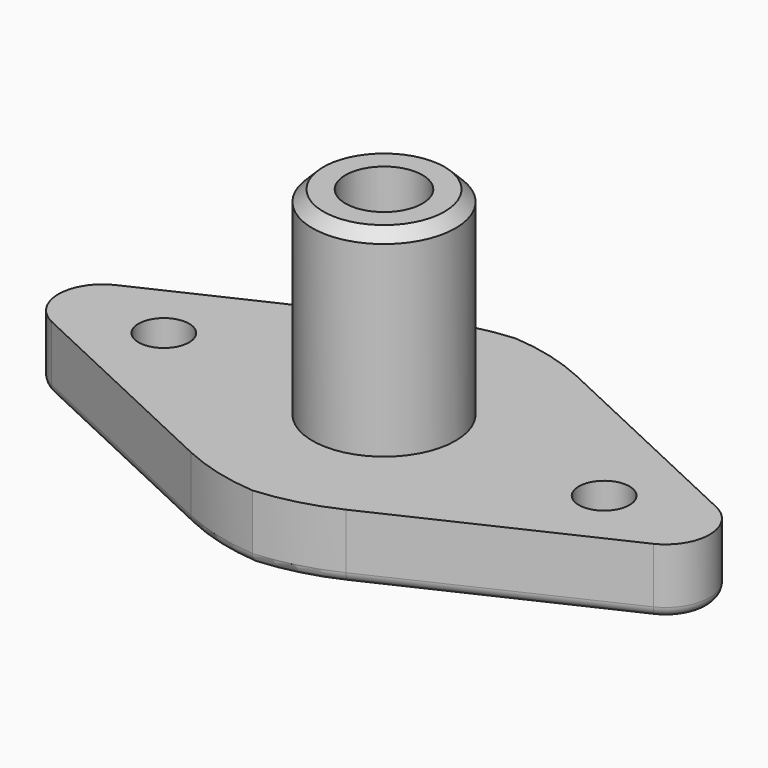
from build123d import *

# Parameters (mm, degrees)
F1_DEPTH      = 3
F2_T1_DEPTH   = 24.3364797517
F3_T1_DEPTH   = 14.1373136471
F4_R          = 3.25
F5_DEPTH      = 9
F6_R          = 1.75
F7_DEPTH      = 12.001
F8_SIZE       = 0.5
F4_R_2        = 1.15
F9_DEPTH      = 3.001
F10_SIZE      = 1
F11_T1_DEPTH  = 11.2158433332
F11_T3_DEPTH  = 11.2158433332
F11_T5_DEPTH  = 11.2158433332
F11_T7_DEPTH  = 11.2158433332
F11_T10_ANGLE = 127.4788590763
F11_T12_ANGLE = 42.4709850422
F11_T14_ANGLE = 42.4709850422
F11_T16_ANGLE = 42.4709850422
F11_T18_ANGLE = 42.4709850422
F11_T20_ANGLE = 127.4788590763


# Not quite as in the source:
# - a fillet or chamfer that OpenCascade refuses, or shapes differently, is made with other operations: its cross-section is extruded or revolved along the edge and cut away or added


with BuildPart() as f1:
    # F0 (on Top) → F1 (new body)
    with BuildSketch(Plane.XY):
        Polygon((-1.5, 7.5), (-17.5, 0), (-1.5, -7.5), (1.5, -7.5), (17.5, 0), (1.5, 7.5), align=None)
    extrude(amount=F1_DEPTH)

    # F2: fillet of radius 2 on 2 edges, made by hand

    # F2_s2 → F2_t1 (cut)
    with BuildSketch(Plane.XY.offset(-10.6682398759)):
        with BuildLine():
            ThreePointArc((-13.6363085399, 1.8115471368), (-14.7878407874, 0), (-13.6363085399, -1.8115471368))
            Line((-13.6363085399, -1.8115471368), (-13.7212248119, -1.9927018505))
            ThreePointArc((-13.7212248119, -1.9927018505), (-15.6529856552, -1.0867471903), (-17.584916272, -0.1811547137))
            Line((-17.584916272, -0.1811547137), (-17.584916272, 0.1811547137))
            ThreePointArc((-17.584916272, 0.1811547137), (-15.6529856552, 1.0867471903), (-13.7212248119, 1.9927018505))
            Line((-13.7212248119, 1.9927018505), (-13.6363085399, 1.8115471368))
        make_face()
        with BuildLine():
            ThreePointArc((13.6363085399, -1.8115471368), (14.7878407874, 0), (13.6363085399, 1.8115471368))
            Line((13.6363085399, 1.8115471368), (13.7212248119, 1.9927018505))
            ThreePointArc((13.7212248119, 1.9927018505), (15.6529856552, 1.0867471903), (17.584916272, 0.1811547137))
            Line((17.584916272, 0.1811547137), (17.584916272, -0.1811547137))
            ThreePointArc((17.584916272, -0.1811547137), (15.6529856552, -1.0867471903), (13.7212248119, -1.9927018505))
            Line((13.7212248119, -1.9927018505), (13.6363085399, -1.8115471368))
        make_face()
    extrude(amount=F2_T1_DEPTH, mode=Mode.SUBTRACT)

    # F3: fillet of radius 10 on 4 edges, made by hand

    # F3_s2 → F3_t1 (cut)
    with BuildSketch(Plane.XY.offset(-5.5686568236)):
        with BuildLine():
            ThreePointArc((-3.5168760329, 6.5545893596), (-1.4467160125, 7.2607861772), (0.7274627294, 7.5))
            Line((0.7274627294, 7.5), (-1.5, 7.5))
            Line((-1.5, 7.5), (-3.5168760329, 6.5545893596))
        make_face()
        with BuildLine():
            ThreePointArc((-0.7274627294, 7.5), (1.4467160125, 7.2607861772), (3.5168760329, 6.5545893596))
            Line((3.5168760329, 6.5545893596), (1.5, 7.5))
            Line((1.5, 7.5), (-0.7274627294, 7.5))
        make_face()
        with BuildLine():
            ThreePointArc((3.5168760329, -6.5545893596), (1.4467160125, -7.2607861772), (-0.7274627294, -7.5))
            Line((-0.7274627294, -7.5), (1.5, -7.5))
            Line((1.5, -7.5), (3.5168760329, -6.5545893596))
        make_face()
        with BuildLine():
            ThreePointArc((0.7274627294, -7.5), (-1.4467160125, -7.2607861772), (-3.5168760329, -6.5545893596))
            Line((-3.5168760329, -6.5545893596), (-1.5, -7.5))
            Line((-1.5, -7.5), (0.7274627294, -7.5))
        make_face()
    extrude(amount=F3_T1_DEPTH, mode=Mode.SUBTRACT)

    # F4 (on face) → F5 (join)
    with BuildSketch(Plane.XY.offset(3)):
        Circle(F4_R)
    extrude(amount=F5_DEPTH)

    # F6 (on face) → F7 (cut, through all)
    with BuildSketch(Plane.XY.offset(12)):
        Circle(F6_R)
    extrude(amount=-F7_DEPTH, mode=Mode.SUBTRACT)

    # F8
    f8_edges = [f1.edges().sort_by_distance(p)[0] for p in [
        (-3.25, 0, 12),
    ]]
    chamfer(f8_edges, length=F8_SIZE)

    # F4 (on face) → F9 (cut, through all)
    with BuildSketch(Plane.XY.offset(3)):
        with Locations((-10, 0)):
            Circle(F4_R_2)
        with Locations((10, 0)):
            Circle(F4_R_2)
    extrude(amount=-F9_DEPTH, mode=Mode.SUBTRACT)

    # F10
    f10_edges = [f1.edges().sort_by_distance(p)[0] for p in [
        (-11.15, 0, 0),
        (8.85, 0, 0),
    ]]
    chamfer(f10_edges, length=F10_SIZE)

    # F11: fillet of radius 0.5 on 10 edges, made by hand

    # F11_s2 → F11_t1 (cut)
    with BuildSketch(Plane(origin=(-10.5198395857, 4.9311748058, 0), x_dir=(0, 0, 1), z_dir=(0.905458936, -0.4244338762, 0))):
        with BuildLine():
            ThreePointArc((-0.0004, 6.9266271486), (0.1464466094, 7.2811462246), (0.5009656854, 7.427992834))
            Line((0.5009656854, 7.427992834), (0.5009656854, 7.4781294026))
            ThreePointArc((0.5009656854, 7.4781294026), (0.2504828427, 7.4777294026), (0, 7.4777294026))
            Line((0, 7.4777294026), (-0.0501365685, 7.427592834))
            ThreePointArc((-0.0501365685, 7.427592834), (-0.0501365685, 7.1771099913), (-0.0505365685, 6.9266271486))
            Line((-0.0505365685, 6.9266271486), (-0.0004, 6.9266271486))
        make_face()
    extrude(amount=F11_T1_DEPTH, mode=Mode.SUBTRACT)

    # F11_s4 → F11_t3 (cut)
    with BuildSketch(Plane(origin=(0.3643540153, 0.1707909447, 0), x_dir=(0, 0, 1), z_dir=(0.905458936, 0.4244338762, 0))):
        with BuildLine():
            ThreePointArc((-0.0004, 6.9266271486), (0.1464466094, 7.2811462246), (0.5009656854, 7.427992834))
            Line((0.5009656854, 7.427992834), (0.5009656854, 7.4781294026))
            ThreePointArc((0.5009656854, 7.4781294026), (0.2504828427, 7.4777294026), (0, 7.4777294026))
            Line((0, 7.4777294026), (-0.0501365685, 7.427592834))
            ThreePointArc((-0.0501365685, 7.427592834), (-0.0501365685, 7.1771099913), (-0.0505365685, 6.9266271486))
            Line((-0.0505365685, 6.9266271486), (-0.0004, 6.9266271486))
        make_face()
    extrude(amount=F11_T3_DEPTH, mode=Mode.SUBTRACT)

    # F11_s6 → F11_t5 (cut)
    with BuildSketch(Plane(origin=(10.5198395857, -4.9311748058, 0), x_dir=(0, 0, 1), z_dir=(-0.905458936, 0.4244338762, 0))):
        with BuildLine():
            ThreePointArc((-0.0004, 6.9266271486), (0.1464466094, 7.2811462246), (0.5009656854, 7.427992834))
            Line((0.5009656854, 7.427992834), (0.5009656854, 7.4781294026))
            ThreePointArc((0.5009656854, 7.4781294026), (0.2504828427, 7.4777294026), (0, 7.4777294026))
            Line((0, 7.4777294026), (-0.0501365685, 7.427592834))
            ThreePointArc((-0.0501365685, 7.427592834), (-0.0501365685, 7.1771099913), (-0.0505365685, 6.9266271486))
            Line((-0.0505365685, 6.9266271486), (-0.0004, 6.9266271486))
        make_face()
    extrude(amount=F11_T5_DEPTH, mode=Mode.SUBTRACT)

    # F11_s8 → F11_t7 (cut)
    with BuildSketch(Plane(origin=(-0.3643540153, -0.1707909447, 0), x_dir=(0, 0, 1), z_dir=(-0.905458936, -0.4244338762, 0))):
        with BuildLine():
            ThreePointArc((-0.0004, 6.9266271486), (0.1464466094, 7.2811462246), (0.5009656854, 7.427992834))
            Line((0.5009656854, 7.427992834), (0.5009656854, 7.4781294026))
            ThreePointArc((0.5009656854, 7.4781294026), (0.2504828427, 7.4777294026), (0, 7.4777294026))
            Line((0, 7.4777294026), (-0.0501365685, 7.427592834))
            ThreePointArc((-0.0501365685, 7.427592834), (-0.0501365685, 7.1771099913), (-0.0505365685, 6.9266271486))
            Line((-0.0505365685, 6.9266271486), (-0.0004, 6.9266271486))
        make_face()
    extrude(amount=F11_T7_DEPTH, mode=Mode.SUBTRACT)

    # F11_s9 → F11_t10 (revolve, cut)
    with BuildSketch(Plane(origin=(10.283861632, -5.0737982035, 0), x_dir=(0, 0, 1), z_dir=(-0.8967911287, 0.4424541462, 0))):
        with BuildLine():
            ThreePointArc((-0.0004, 7.157454968), (0.1464466094, 7.511974044), (0.5009656854, 7.6588206534))
            Line((0.5009656854, 7.6588206534), (0.5009656854, 7.708957222))
            ThreePointArc((0.5009656854, 7.708957222), (0.2504828427, 7.708557222), (0, 7.708557222))
            Line((0, 7.708557222), (-0.0501365685, 7.6584206534))
            ThreePointArc((-0.0501365685, 7.6584206534), (-0.0501365685, 7.4079378107), (-0.0505365685, 7.157454968))
            Line((-0.0505365685, 7.157454968), (-0.0004, 7.157454968))
        make_face()
    revolve(axis=Axis((12.7871458195, 0, 0), (0, 0, -1)), revolution_arc=F11_T10_ANGLE, mode=Mode.SUBTRACT)

    # F11_s11 → F11_t12 (revolve, cut)
    with BuildSketch(Plane(origin=(-1.3745464916, -0.429601751, 0), x_dir=(0, 0, 1), z_dir=(-0.9544689122, -0.2983104016, 0))):
        with BuildLine():
            ThreePointArc((-0.0004, 7.3298717335), (0.1464466094, 7.6843908095), (0.5009656854, 7.8312374189))
            Line((0.5009656854, 7.8312374189), (0.5009656854, 7.8813739874))
            ThreePointArc((0.5009656854, 7.8813739874), (0.2504828427, 7.8809739874), (0, 7.8809739874))
            Line((0, 7.8809739874), (-0.0501365685, 7.8308374189))
            ThreePointArc((-0.0501365685, 7.8308374189), (-0.0501365685, 7.5803545762), (-0.0505365685, 7.3298717335))
            Line((-0.0505365685, 7.3298717335), (-0.0004, 7.3298717335))
        make_face()
    revolve(axis=Axis((-0.72746273, -2.5000000027, 0), (0, 0, -1)), revolution_arc=F11_T12_ANGLE, mode=Mode.SUBTRACT)

    # F11_s13 → F11_t14 (revolve, cut)
    with BuildSketch(Plane(origin=(-0.3643540157, -0.1707909448, 0), x_dir=(0, 0, 1), z_dir=(-0.905458936, -0.4244338762, 0))):
        with BuildLine():
            ThreePointArc((-0.0004, 6.9266271486), (0.1464466094, 7.2811462246), (0.5009656854, 7.427992834))
            Line((0.5009656854, 7.427992834), (0.5009656854, 7.4781294026))
            ThreePointArc((0.5009656854, 7.4781294026), (0.2504828427, 7.4777294026), (0, 7.4777294026))
            Line((0, 7.4777294026), (-0.0501365685, 7.427592834))
            ThreePointArc((-0.0501365685, 7.427592834), (-0.0501365685, 7.1771099913), (-0.0505365685, 6.9266271486))
            Line((-0.0505365685, 6.9266271486), (-0.0004, 6.9266271486))
        make_face()
    revolve(axis=Axis((0.72746273, -2.5000000027, 0), (0, 0, -1)), revolution_arc=F11_T14_ANGLE, mode=Mode.SUBTRACT)

    # F11_s15 → F11_t16 (revolve, cut)
    with BuildSketch(Plane(origin=(0.3643540157, 0.1707909448, 0), x_dir=(0, 0, 1), z_dir=(0.905458936, 0.4244338762, 0))):
        with BuildLine():
            ThreePointArc((-0.0004, 6.9266271486), (0.1464466094, 7.2811462246), (0.5009656854, 7.427992834))
            Line((0.5009656854, 7.427992834), (0.5009656854, 7.4781294026))
            ThreePointArc((0.5009656854, 7.4781294026), (0.2504828427, 7.4777294026), (0, 7.4777294026))
            Line((0, 7.4777294026), (-0.0501365685, 7.427592834))
            ThreePointArc((-0.0501365685, 7.427592834), (-0.0501365685, 7.1771099913), (-0.0505365685, 6.9266271486))
            Line((-0.0505365685, 6.9266271486), (-0.0004, 6.9266271486))
        make_face()
    revolve(axis=Axis((-0.72746273, 2.5000000027, 0), (0, 0, -1)), revolution_arc=F11_T16_ANGLE, mode=Mode.SUBTRACT)

    # F11_s17 → F11_t18 (revolve, cut)
    with BuildSketch(Plane(origin=(1.3745464916, 0.429601751, 0), x_dir=(0, 0, 1), z_dir=(0.9544689122, 0.2983104016, 0))):
        with BuildLine():
            ThreePointArc((-0.0004, 7.3298717335), (0.1464466094, 7.6843908095), (0.5009656854, 7.8312374189))
            Line((0.5009656854, 7.8312374189), (0.5009656854, 7.8813739874))
            ThreePointArc((0.5009656854, 7.8813739874), (0.2504828427, 7.8809739874), (0, 7.8809739874))
            Line((0, 7.8809739874), (-0.0501365685, 7.8308374189))
            ThreePointArc((-0.0501365685, 7.8308374189), (-0.0501365685, 7.5803545762), (-0.0505365685, 7.3298717335))
            Line((-0.0505365685, 7.3298717335), (-0.0004, 7.3298717335))
        make_face()
    revolve(axis=Axis((0.72746273, 2.5000000027, 0), (0, 0, -1)), revolution_arc=F11_T18_ANGLE, mode=Mode.SUBTRACT)

    # F11_s19 → F11_t20 (revolve, cut)
    with BuildSketch(Plane(origin=(-10.283861632, 5.0737982035, 0), x_dir=(0, 0, 1), z_dir=(0.8967911287, -0.4424541462, 0))):
        with BuildLine():
            ThreePointArc((-0.0004, 7.157454968), (0.1464466094, 7.511974044), (0.5009656854, 7.6588206534))
            Line((0.5009656854, 7.6588206534), (0.5009656854, 7.708957222))
            ThreePointArc((0.5009656854, 7.708957222), (0.2504828427, 7.708557222), (0, 7.708557222))
            Line((0, 7.708557222), (-0.0501365685, 7.6584206534))
            ThreePointArc((-0.0501365685, 7.6584206534), (-0.0501365685, 7.4079378107), (-0.0505365685, 7.157454968))
            Line((-0.0505365685, 7.157454968), (-0.0004, 7.157454968))
        make_face()
    revolve(axis=Axis((-12.7871458195, 0, 0), (0, 0, -1)), revolution_arc=F11_T20_ANGLE, mode=Mode.SUBTRACT)


solid = f1.part
